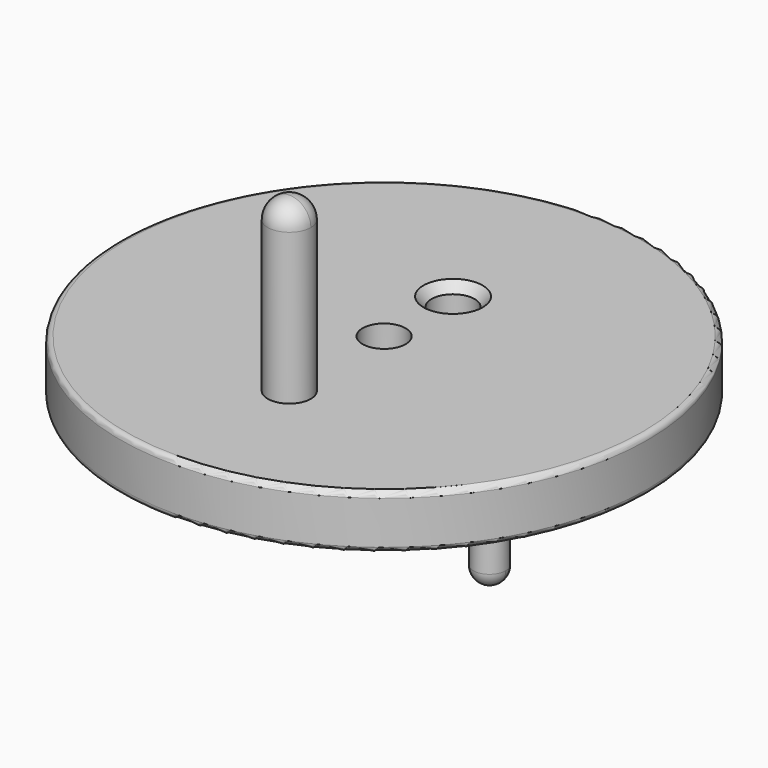
from build123d import *

# Parameters (mm, degrees)
F0_R           = 38.89375
F0_R_2         = 3.175
F1_DEPTH       = 7.9375
F2_DEPTH       = 30.1625
F4_ANGLE       = 180
F6_D           = 6.35
F6_CSINK_D     = 8.7376
F6_CSINK_ANGLE = 82
F7_R           = 26.19375
F7_R_2         = 3.175
F8_DEPTH       = 0.7874
F7_R_3         = 2.38125
F9_DEPTH       = 5.5499
F13_ANGLE      = 180
F14_ANGLE      = 180
F15_ANGLE      = 180
F16_R          = 0.7874


with BuildPart() as f1:
    # F0 (on Top) → F1 (new body)
    with BuildSketch(Plane.XY):
        Circle(F0_R)
        with Locations((0, -17.4625)):
            Circle(F0_R_2, mode=Mode.SUBTRACT)
        Circle(F0_R_2, mode=Mode.SUBTRACT)
    extrude(amount=F1_DEPTH)

    # F0 (on Top) → F2 (join)
    with BuildSketch(Plane.XY):
        with Locations((0, -17.4625)):
            Circle(F0_R_2)
    extrude(amount=F2_DEPTH)

    # F3 (on face) → F4 (revolve)
    with BuildSketch(Plane.XY.offset(30.1625)):
        with BuildLine():
            ThreePointArc((3.175, -17.4625), (2.2450640303, -15.2174359697), (0, -14.2875))
            Line((0, -14.2875), (0, -20.6375))
            ThreePointArc((0, -20.6375), (2.2450640303, -19.7075640303), (3.175, -17.4625))
        make_face()
    revolve(axis=Axis((0, -17.4625, 30.1625), (0, -1, 0)), revolution_arc=F4_ANGLE)

    # F6 (through all)
    with Locations(Plane.XY.offset(7.9375)):
        with Locations((0, 12.7)):
            CounterSinkHole(F6_D / 2, F6_CSINK_D / 2, counter_sink_angle=F6_CSINK_ANGLE)

    # F7 (on face) → F8 (cut)
    with BuildSketch(Plane(origin=(0, 0, 0), x_dir=(1, 0, 0), z_dir=(0, 0, -1))):
        Circle(F7_R)
        with Locations((0, -12.7)):
            Circle(F7_R_2, mode=Mode.SUBTRACT)
        Circle(F7_R_2, mode=Mode.SUBTRACT)
    extrude(amount=-F8_DEPTH, mode=Mode.SUBTRACT)

    # F7 (on face) → F9 (join)
    with BuildSketch(Plane(origin=(0, 0, 0), x_dir=(1, 0, 0), z_dir=(0, 0, -1))):
        with Locations((0, -33.3375)):
            Circle(F7_R_3)
        with Locations((-28.8711218987, 16.66875)):
            Circle(F7_R_3)
        with Locations((28.8711218987, 16.66875)):
            Circle(F7_R_3)
    extrude(amount=F9_DEPTH)

    # F12 (on face) → F13 (revolve)
    with BuildSketch(Plane(origin=(0, 0, -5.5499), x_dir=(1, 0, 0), z_dir=(0, 0, -1))):
        with BuildLine():
            Line((0, -30.95625), (0, -33.3375))
            Line((0, -33.3375), (0, -35.71875))
            ThreePointArc((0, -35.71875), (1.6837980227, -35.0212980227), (2.38125, -33.3375))
            ThreePointArc((2.38125, -33.3375), (1.6837980227, -31.6537019773), (0, -30.95625))
        make_face()
    revolve(axis=Axis((0, 33.3375, -5.5499), (0, 1, 0)), revolution_arc=F13_ANGLE)

    # F11 (on face) → F14 (revolve)
    with BuildSketch(Plane(origin=(0, 0, -5.5499), x_dir=(1, 0, 0), z_dir=(0, 0, -1))):
        with BuildLine():
            Line((28.8711218987, 19.05), (28.8711218987, 16.66875))
            Line((28.8711218987, 16.66875), (28.8711218987, 14.2875))
            ThreePointArc((28.8711218987, 14.2875), (30.5549199214, 14.9849519773), (31.2523718987, 16.66875))
            ThreePointArc((31.2523718987, 16.66875), (30.5549199214, 18.3525480227), (28.8711218987, 19.05))
        make_face()
    revolve(axis=Axis((28.8711218987, -16.66875, -5.5499), (0, 1, 0)), revolution_arc=F14_ANGLE)

    # F10 (on face) → F15 (revolve)
    with BuildSketch(Plane(origin=(0, 0, -5.5499), x_dir=(1, 0, 0), z_dir=(0, 0, -1))):
        with BuildLine():
            Line((-28.8711218987, 19.05), (-28.8711218987, 16.66875))
            Line((-28.8711218987, 16.66875), (-28.8711218987, 14.2875))
            ThreePointArc((-28.8711218987, 14.2875), (-27.187323876, 14.9849519773), (-26.4898718987, 16.66875))
            ThreePointArc((-26.4898718987, 16.66875), (-27.187323876, 18.3525480227), (-28.8711218987, 19.05))
        make_face()
    revolve(axis=Axis((-28.8711218987, -16.66875, -5.5499), (0, 1, 0)), revolution_arc=F15_ANGLE)

    # F16
    f16_edges = [f1.edges().sort_by_distance(p)[0] for p in [
        (-38.89375, 0, 7.9375),
        (-38.89375, 0, 0),
    ]]
    fillet(f16_edges, radius=F16_R)


solid = f1.part
